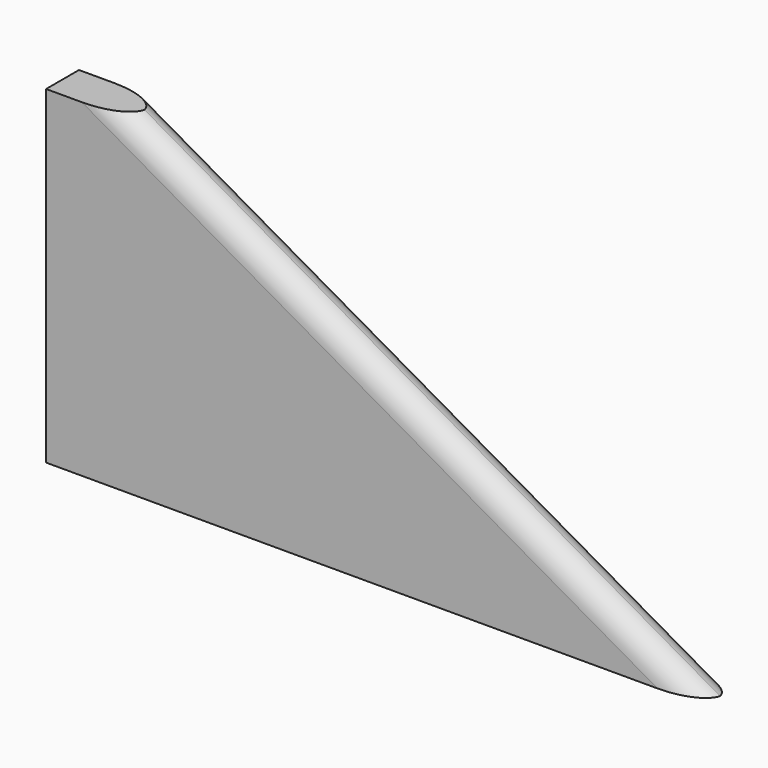
from build123d import *

# Parameters (mm, degrees)
F1_DEPTH    = 3.175
F2_T1_DEPTH = 60.0853367017


# Not quite as in the source:
# - a fillet or chamfer that OpenCascade refuses, or shapes differently, is made with other operations: its cross-section is extruded or revolved along the edge and cut away or added


with BuildPart() as f1:
    # F0 (on Front) → F1 (new body)
    with BuildSketch(Plane.XZ):
        Polygon((0, 25.4), (0, 0), (50.8, 0), (6.35, 25.4), align=None)
    extrude(amount=F1_DEPTH)

    # F2: fillet of radius 1.778 on 2 edges, made by hand

    # F2_s2 → F2_t1 (cut)
    with BuildSketch(Plane(origin=(42.1547253821, 0, -24.0884145041), x_dir=(0, 1, 0), z_dir=(-0.8682431421, 0, 0.4961389384))):
        with BuildLine():
            ThreePointArc((-1.397, -25.2038580685), (-2.6542358569, -24.6830939255), (-3.175, -23.4258580685))
            Line((-3.175, -23.4258580685), (-3.175, -25.2038580685))
            Line((-3.175, -25.2038580685), (-1.397, -25.2038580685))
        make_face()
        with BuildLine():
            ThreePointArc((-1.778, -25.2038580685), (-0.5207641431, -24.6830939255), (0, -23.4258580685))
            Line((0, -23.4258580685), (0, -25.2038580685))
            Line((0, -25.2038580685), (-1.778, -25.2038580685))
        make_face()
    extrude(amount=F2_T1_DEPTH, mode=Mode.SUBTRACT)


solid = f1.part
